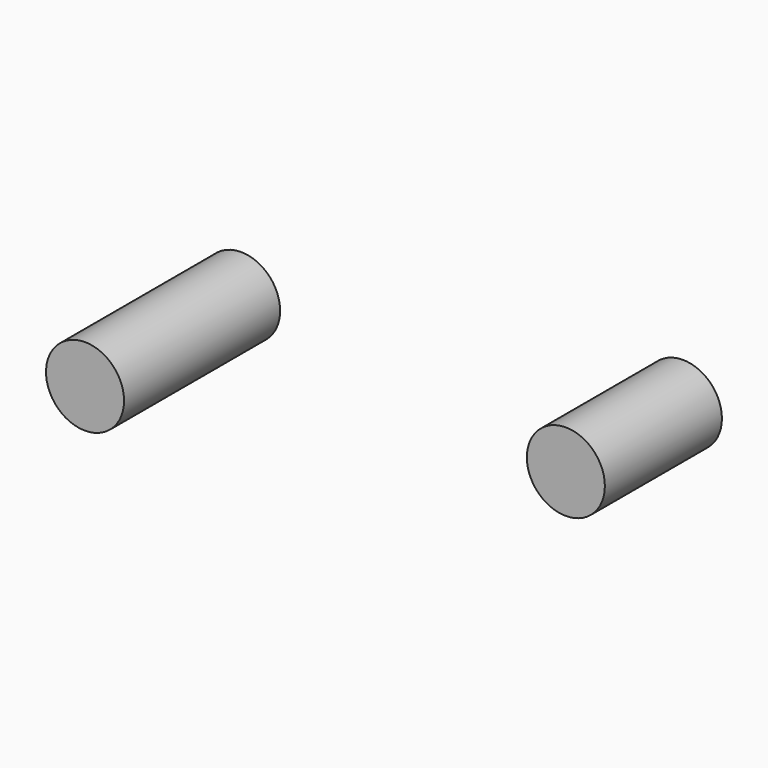
from build123d import *

# Parameters (mm, degrees)
F2_R     = 2
F3_DEPTH = 3.75
F4_R     = 2
F5_DEPTH = 10


with BuildPart() as f3:
    # F2 (on Front) → F3 (new body, symmetric)
    with BuildSketch(Plane.XZ):
        Circle(F2_R)
    extrude(amount=F3_DEPTH, both=True)


with BuildPart() as f5:
    # F4 (on Front) → F5 (new body)
    with BuildSketch(Plane.XZ):
        with Locations((-19.6472983807, 0)):
            Circle(F4_R)
    extrude(amount=F5_DEPTH)


solid = Compound([f3.part, f5.part])
